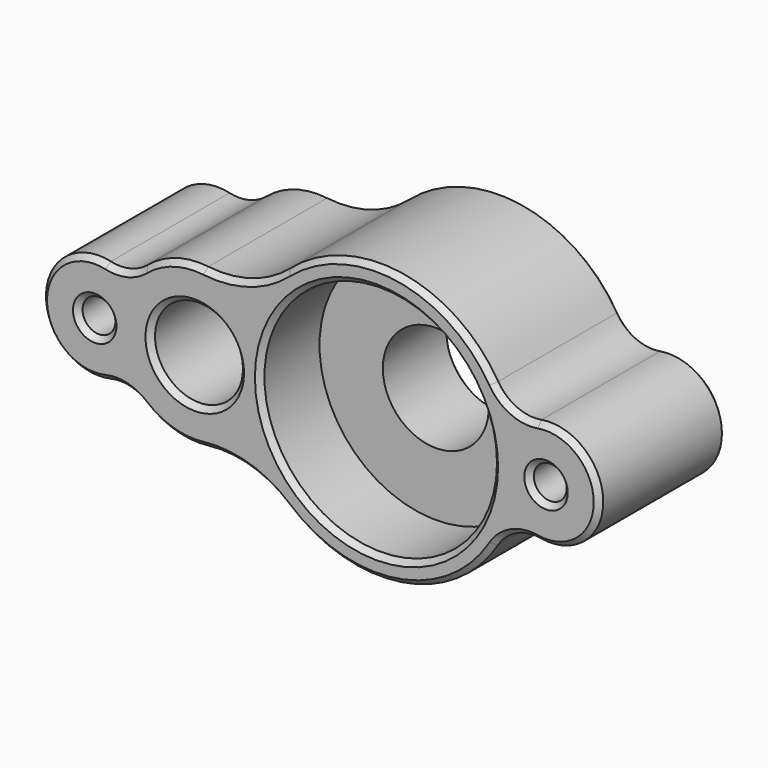
from build123d import *

# Parameters (mm, degrees)
F1_R     = 1.5499996566
F1_R_2   = 4.15
F1_R_3   = 10.975
F2_DEPTH = 15
F3_R     = 1.5499996566
F3_R_2   = 10.975
F3_R_3   = 4.15
F3_R_4   = 5
F4_DEPTH = 8
F5_SIZE  = 0.5


# Not quite as in the source:
# - a feature names something its author has since deleted; it is built from what else it names


with BuildPart() as f2:
    # F1 (on offset) → F2 (new body)
    with BuildSketch(Plane.XZ.offset(7.5)):
        with BuildLine():
            ThreePointArc((-16.6892397333, 5.7083826769), (-18.3305665894, 4.8749174948), (-20.1713586703, 4.8647896648))
            ThreePointArc((-20.1713586703, 4.8647896648), (-26.2950827169, -0.0072979827), (-20.1713596113, -4.879386813))
            ThreePointArc((-20.1713596113, -4.879386813), (-18.3305675322, -4.8895149984), (-16.6892408371, -5.7229804975))
            ThreePointArc((-16.6892408371, -5.7229804975), (-14.008426037, -7.1768258733), (-10.9702112996, -7.4408061354))
            ThreePointArc((-10.9702112996, -7.4408061354), (-6.8485397196, -7.8126278343), (-3.2303605207, -9.8214103693))
            ThreePointArc((-3.2303605207, -9.8214103693), (7.2785660743, -12.855093715), (16.3833205976, -6.7933928076))
            ThreePointArc((16.3833205976, -6.7933928076), (18.1382514389, -5.2406931628), (20.4617514792, -4.9373682419))
            ThreePointArc((20.4617514792, -4.9373682419), (26.2950863861, -0.0073004118), (20.4617519197, 4.9227679396))
            ThreePointArc((20.4617519197, 4.9227679396), (18.1382519066, 5.2260930681), (16.383321204, 6.7787928697))
            ThreePointArc((16.383321204, 6.7787928697), (7.2785667206, 12.8404946682), (-3.2303604104, 9.8068115182))
            ThreePointArc((-3.2303604104, 9.8068115182), (-6.8485396319, 7.7980290238), (-10.970211216, 7.4262073712))
            ThreePointArc((-10.970211216, 7.4262073712), (-14.0084253044, 7.1622273392), (-16.6892397333, 5.7083826769))
        make_face()
        with Locations((21.2950848365, -0.0073001884)):
            Circle(F1_R, mode=Mode.SUBTRACT)
        with Locations((-21.2950828407, -0.0072984656)):
            Circle(F1_R, mode=Mode.SUBTRACT)
        with Locations((-11.8549144411, -0.0072993771)):
            Circle(F1_R_2, mode=Mode.SUBTRACT)
        with Locations((5.2950859535, -0.0072994735)):
            Circle(F1_R_3, mode=Mode.SUBTRACT)
    extrude(amount=-F2_DEPTH)

    # F3 (on face) → F4 (join)
    with BuildSketch(Plane(origin=(0, 7.5, 0), x_dir=(-1, 0, 0), z_dir=(0, 1, 0))):
        with BuildLine():
            ThreePointArc((10.970211216, 7.4262073712), (6.8485396319, 7.7980290238), (3.2303604104, 9.8068115182))
            ThreePointArc((3.2303604104, 9.8068115182), (-7.2785667206, 12.8404946682), (-16.383321204, 6.7787928697))
            ThreePointArc((-16.383321204, 6.7787928697), (-18.1382519066, 5.2260930681), (-20.4617519197, 4.9227679396))
            ThreePointArc((-20.4617519197, 4.9227679396), (-26.2950863861, -0.0073004118), (-20.4617514792, -4.9373682419))
            ThreePointArc((-20.4617514792, -4.9373682419), (-18.1382514389, -5.2406931628), (-16.3833205976, -6.7933928076))
            ThreePointArc((-16.3833205976, -6.7933928076), (-7.2785660743, -12.855093715), (3.2303605207, -9.8214103693))
            ThreePointArc((3.2303605207, -9.8214103693), (6.8485397196, -7.8126278343), (10.9702112996, -7.4408061354))
            ThreePointArc((10.9702112996, -7.4408061354), (14.008426037, -7.1768258733), (16.6892408371, -5.7229804975))
            ThreePointArc((16.6892408371, -5.7229804975), (18.3305675322, -4.8895149984), (20.1713596113, -4.879386813))
            ThreePointArc((20.1713596113, -4.879386813), (26.2950827169, -0.0072979827), (20.1713586703, 4.8647896648))
            ThreePointArc((20.1713586703, 4.8647896648), (18.3305665894, 4.8749174948), (16.6892397333, 5.7083826769))
            ThreePointArc((16.6892397333, 5.7083826769), (14.0084253044, 7.1622273392), (10.970211216, 7.4262073712))
        make_face()
        with Locations((-21.2950848365, -0.0073001884)):
            Circle(F3_R, mode=Mode.SUBTRACT)
        with Locations((-5.2950859535, -0.0072994735)):
            Circle(F3_R_2, mode=Mode.SUBTRACT)
        with Locations((11.8549144411, -0.0072993771)):
            Circle(F3_R_3, mode=Mode.SUBTRACT)
        with Locations((21.2950828407, -0.0072984656)):
            Circle(F3_R, mode=Mode.SUBTRACT)
        with Locations((-5.2950859535, -0.0072994735)):
            Circle(F3_R_2)
        with Locations((-5.2950859535, -0.0072994735)):
            Circle(F3_R_4, mode=Mode.SUBTRACT)
    extrude(amount=-F4_DEPTH)

    # F5
    f5_edges = [f2.edges().sort_by_distance(p)[0] for p in [
        (-6.84854, -7.5, 7.798029),
        (7.278567, -7.5, 12.840495),
        (18.138252, -7.5, 5.226093),
        (26.295086, -7.5, -0.0073),
        (18.138251, -7.5, -5.240693),
        (7.278566, -7.5, -12.855094),
        (-6.84854, -7.5, -7.812628),
        (-14.008426, -7.5, -7.176826),
        (-18.330568, -7.5, -4.889515),
        (-26.295083, -7.5, -0.007298),
        (-18.330567, -7.5, 4.874917),
        (-14.008425, -7.5, 7.162227),
        (-5.679914, -7.5, -0.007299),
        (-22.845082, -7.5, -0.007298),
        (19.745085, -7.5, -0.0073),
        (7.278567, 7.5, 12.840495),
        (-22.845082, 7.5, -0.007298),
        (10.295086, 7.5, -0.007299),
        (19.745085, 7.5, -0.0073),
        (-16.004914, -7.5, -0.007299),
        (-6.84854, 7.5, 7.798029),
        (-14.008425, 7.5, 7.162227),
        (-18.330567, 7.5, 4.874917),
        (-26.295083, 7.5, -0.007298),
        (-18.330568, 7.5, -4.889515),
        (-14.008426, 7.5, -7.176826),
        (-6.84854, 7.5, -7.812628),
        (7.278566, 7.5, -12.855094),
        (18.138251, 7.5, -5.240693),
        (26.295086, 7.5, -0.0073),
        (18.138252, 7.5, 5.226093),
    ]]
    chamfer(f5_edges, length=F5_SIZE)


solid = f2.part
